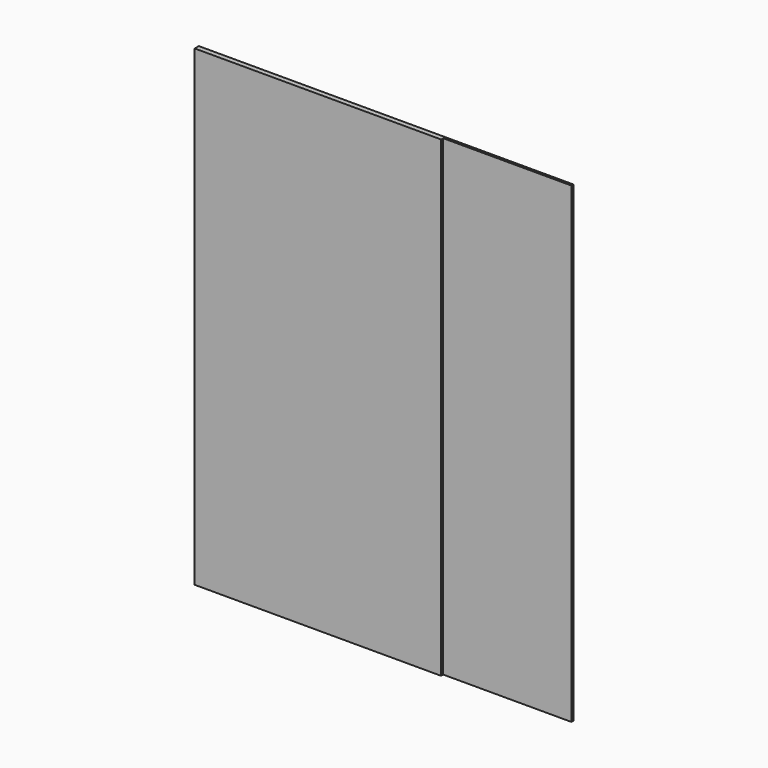
from build123d import *

# Parameters (mm, degrees)
F0_W     = 45
F0_H     = 2060
F0_W_2   = 22.5
F1_DEPTH = 50
F0_W_3   = 499.5
F2_DEPTH = 12
F0_W_4   = 531
F3_DEPTH = 25


# Not quite as in the source:
# - a feature names something its author has since deleted; it is built from what else it names


with BuildPart() as f1:
    # F0 (on Front) → F1 (new body)
    with BuildSketch(Plane.XZ):
        with Locations((832.5, 0)):
            Rectangle(F0_W, F0_H)
        Polygon((288, -1075), (855, -1075), (855, -1030), (810, -1030), (310.5, -1030), (288, -1030), align=None)
        Polygon((-855, -1075), (288, -1075), (288, -1030), (265.5, -1030), (-265.5, -1030), (-310.5, -1030), (-810, -1030), (-855, -1030), align=None)
        with Locations((-832.5, 0)):
            Rectangle(F0_W, F0_H)
        with Locations((276.75, 0)):
            Rectangle(F0_W_2, F0_H)
        Polygon((810, 1030), (855, 1030), (855, 1075), (288, 1075), (288, 1030), (310.5, 1030), align=None)
        Polygon((265.5, 1030), (288, 1030), (288, 1075), (-855, 1075), (-855, 1030), (-810, 1030), (-310.5, 1030), (-265.5, 1030), align=None)
        with Locations((-288, 0)):
            Rectangle(F0_W, F0_H)
        with Locations((299.25, 0)):
            Rectangle(F0_W_2, F0_H)
    extrude(amount=-F1_DEPTH)

    # F0 (on Front) → F2 (join)
    with BuildSketch(Plane.XZ):
        Polygon((855, -1030), (855, -1075), (288, -1075), (288, -1125), (912, -1125), (912, 1175), (288, 1175), (288, 1075), (855, 1075), (855, 1030), align=None)
        with Locations((560.25, 0)):
            Rectangle(F0_W_3, F0_H)
        Polygon((288, -1075), (855, -1075), (855, -1030), (810, -1030), (310.5, -1030), (288, -1030), align=None)
        with Locations((832.5, 0)):
            Rectangle(F0_W, F0_H)
        Polygon((810, 1030), (855, 1030), (855, 1075), (288, 1075), (288, 1030), (310.5, 1030), align=None)
        with Locations((299.25, 0)):
            Rectangle(F0_W_2, F0_H)
    extrude(amount=F2_DEPTH)

    # F0 (on Front) → F3 (join)
    with BuildSketch(Plane.XZ):
        Polygon((288, -1125), (288, -1075), (-855, -1075), (-855, -1030), (-855, 1030), (-855, 1075), (288, 1075), (288, 1175), (-912, 1175), (-912, -1125), align=None)
        with Locations((-288, 0)):
            Rectangle(F0_W, F0_H)
        Polygon((265.5, 1030), (288, 1030), (288, 1075), (-855, 1075), (-855, 1030), (-810, 1030), (-310.5, 1030), (-265.5, 1030), align=None)
        with Locations((-832.5, 0)):
            Rectangle(F0_W, F0_H)
        with Locations((-560.25, 0)):
            Rectangle(F0_W_3, F0_H)
        Rectangle(F0_W_4, F0_H)
        Polygon((-855, -1075), (288, -1075), (288, -1030), (265.5, -1030), (-265.5, -1030), (-310.5, -1030), (-810, -1030), (-855, -1030), align=None)
        with Locations((276.75, 0)):
            Rectangle(F0_W_2, F0_H)
    extrude(amount=F3_DEPTH)


solid = f1.part
